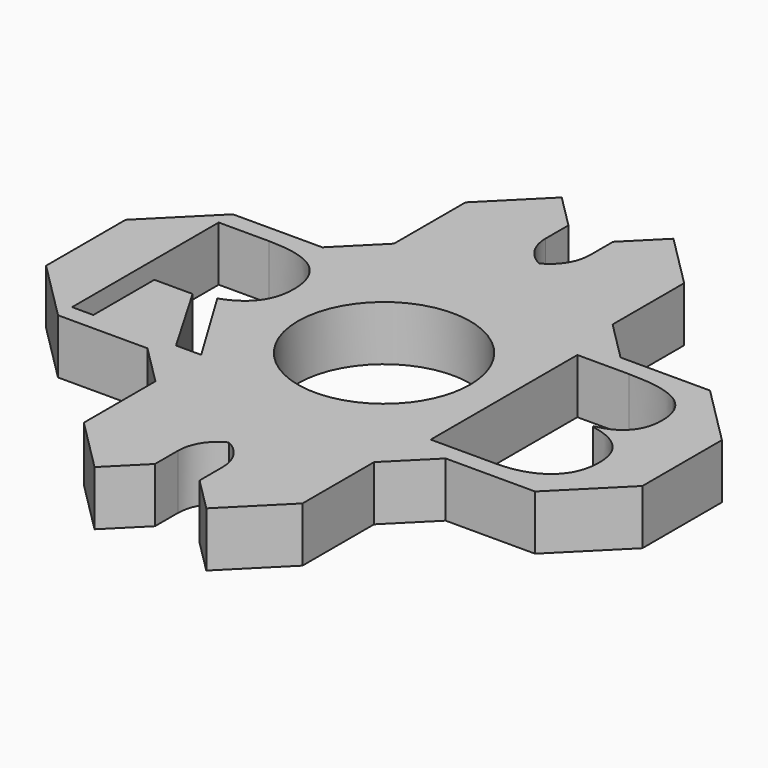
from build123d import *

# Parameters (mm, degrees)
F0_W        = 24.13
F0_H        = 27.94
F0_W_2      = 27.94
F1_DEPTH    = 7
F0_H_2      = 24.13
F2_DEPTH    = 7
F3_SIZE     = 7.62
F4_SIZE     = 5.08
F5_W        = 5.6953141466
F5_H        = 27.5579802692
F5_H_2      = 20.2091857791
F6_DEPTH    = 46.736
F7_T1_DEPTH = 33.1282991577
F8_T1_DEPTH = 7


# Not quite as in the source:
# - a fillet or chamfer that OpenCascade refuses, or shapes differently, is made with other operations: its cross-section is extruded or revolved along the edge and cut away or added


with BuildPart() as f1:
    # F0 (on Top) → F1 (new body)
    with BuildSketch(Plane.XY):
        with Locations((-26.035, 0)):
            Rectangle(F0_W, F0_H)
        with BuildLine():
            Line((-22.8701785602, -1.9821503455), (-27.7604957957, -1.9821503455))
            Line((-27.7604957957, -1.9821503455), (-27.7604957957, -11.721775867))
            Line((-27.7604957957, -11.721775867), (-30.4824648231, -11.721775867))
            Line((-30.4824648231, -11.721775867), (-30.4824648231, 11.6994604529))
            Line((-30.4824648231, 11.6994604529), (-24.0594380975, 11.6994604529))
            add(Edge.make_bspline(
                [(-24.0594380975, 11.6994604529), (-19.7483722746, 11.6994604529), (-17.6902356183, 10.0488502329)],
                knots=[0, 0, 0, 1, 1, 1], degree=2))
            add(Edge.make_bspline(
                [(-17.6902356183, 10.0488502329), (-15.6320989621, 8.398240013), (-15.6320989621, 5.0816412169)],
                knots=[0, 0, 0, 1, 1, 1], degree=2))
            add(Edge.make_bspline(
                [(-15.6320989621, 5.0816412169), (-15.6320989621, 0.4373776788), (-20.3430020433, -1.1978541851)],
                knots=[0, 0, 0, 1, 1, 1], degree=2))
            Line((-20.3430020433, -1.1978541851), (-13.9814887421, -11.721775867))
            Line((-13.9814887421, -11.721775867), (-17.2006912829, -11.721775867))
            Line((-17.2006912829, -11.721775867), (-22.8701785602, -1.9821503455))
        make_face(mode=Mode.SUBTRACT)
        Rectangle(F0_W_2, F0_H)
        with BuildLine():
            ThreePointArc((8.7965986845, 6.6045326545), (10.4346199147, 3.4811933637), (11, 0))
            ThreePointArc((11, 0), (10.4117353498, -3.5490515643), (8.7098605443, -6.7185064783))
            add(Edge.make_bspline(
                [(8.7098605443, -6.7185064783), (8.1189739543, -7.8747447622), (7.281651607, -8.8229557447)],
                knots=[0.7056859188, 0.7056859188, 0.7056859188, 1, 1, 1], degree=2))
            add(Edge.make_bspline(
                [(7.281651607, -8.8229557447), (4.436655731, -12.0447213449), (-0.6228234215, -12.0447213449)],
                knots=[0, 0, 0, 1, 1, 1], degree=2))
            add(Edge.make_bspline(
                [(-0.6228234215, -12.0447213449), (-5.7950771853, -12.0447213449), (-8.6067532898, -8.8793430504)],
                knots=[0, 0, 0, 1, 1, 1], degree=2))
            add(Edge.make_bspline(
                [(-8.6067532898, -8.8793430504), (-11.4184293943, -5.7139647559), (-11.4184293943, 0.0529187766)],
                knots=[0, 0, 0, 1, 1, 1], degree=2))
            add(Edge.make_bspline(
                [(-11.4184293943, 0.0529187766), (-11.4184293943, 5.7736672408), (-8.5990641118, 8.9211041199)],
                knots=[0, 0, 0, 1, 1, 1], degree=2))
            add(Edge.make_bspline(
                [(-8.5990641118, 8.9211041199), (-5.7796988292, 12.068540999), (-0.5920667093, 12.068540999)],
                knots=[0, 0, 0, 1, 1, 1], degree=2))
            add(Edge.make_bspline(
                [(-0.5920667093, 12.068540999), (4.4571602058, 12.068540999), (7.2919038444, 8.8647168143)],
                knots=[0, 0, 0, 1, 1, 1], degree=2))
            add(Edge.make_bspline(
                [(7.2919038444, 8.8647168143), (8.1849092487, 7.8554430753), (8.7965986845, 6.6045326545)],
                knots=[0, 0, 0, 0.3150215745, 0.3150215745, 0.3150215745], degree=2))
        make_face(mode=Mode.SUBTRACT)
        with Locations((26.035, 0)):
            Rectangle(F0_W, F0_H)
        with BuildLine():
            Line((15.3450363151, -11.721775867), (15.3450363151, 11.6994604529))
            Line((15.3450363151, 11.6994604529), (21.9628555511, 11.6994604529))
            add(Edge.make_bspline(
                [(21.9628555511, 11.6994604529), (26.6224974453, 11.6994604529), (28.706264695, 10.3051561677)],
                knots=[0, 0, 0, 1, 1, 1], degree=2))
            add(Edge.make_bspline(
                [(28.706264695, 10.3051561677), (30.7900319448, 8.9108518825), (30.7900319448, 5.9018202082)],
                knots=[0, 0, 0, 1, 1, 1], degree=2))
            add(Edge.make_bspline(
                [(30.7900319448, 5.9018202082), (30.7900319448, 3.8154898992), (29.6289660602, 2.4621945635)],
                knots=[0, 0, 0, 1, 1, 1], degree=2))
            add(Edge.make_bspline(
                [(29.6289660602, 2.4621945635), (28.4679001757, 1.1088992279), (26.2380385431, 0.7090619697)],
                knots=[0, 0, 0, 1, 1, 1], degree=2))
            Line((26.2380385431, 0.7090619697), (26.2380385431, 0.5501522901))
            add(Edge.make_bspline(
                [(26.2380385431, 0.5501522901), (31.5743281052, -0.3622968377), (31.5743281052, -5.0578215628)],
                knots=[0, 0, 0, 1, 1, 1], degree=2))
            add(Edge.make_bspline(
                [(31.5743281052, -5.0578215628), (31.5743281052, -8.1950062045), (29.4521149653, -9.9583910358)],
                knots=[0, 0, 0, 1, 1, 1], degree=2))
            add(Edge.make_bspline(
                [(29.4521149653, -9.9583910358), (27.3299018253, -11.721775867), (23.5160695158, -11.721775867)],
                knots=[0, 0, 0, 1, 1, 1], degree=2))
            Line((23.5160695158, -11.721775867), (15.3450363151, -11.721775867))
        make_face(mode=Mode.SUBTRACT)
        with BuildLine():
            ThreePointArc((8.7098605443, -6.7185064783), (-10.9997668891, 0.0716127389), (8.7965986845, 6.6045326545))
            add(Edge.make_bspline(
                [(7.2919038444, 8.8647168143), (8.1849092487, 7.8554430753), (8.7965986845, 6.6045326545)],
                knots=[0, 0, 0, 0.3150215745, 0.3150215745, 0.3150215745], degree=2))
            add(Edge.make_bspline(
                [(-0.5920667093, 12.068540999), (4.4571602058, 12.068540999), (7.2919038444, 8.8647168143)],
                knots=[0, 0, 0, 1, 1, 1], degree=2))
            add(Edge.make_bspline(
                [(-8.5990641118, 8.9211041199), (-5.7796988292, 12.068540999), (-0.5920667093, 12.068540999)],
                knots=[0, 0, 0, 1, 1, 1], degree=2))
            add(Edge.make_bspline(
                [(-11.4184293943, 0.0529187766), (-11.4184293943, 5.7736672408), (-8.5990641118, 8.9211041199)],
                knots=[0, 0, 0, 1, 1, 1], degree=2))
            add(Edge.make_bspline(
                [(-8.6067532898, -8.8793430504), (-11.4184293943, -5.7139647559), (-11.4184293943, 0.0529187766)],
                knots=[0, 0, 0, 1, 1, 1], degree=2))
            add(Edge.make_bspline(
                [(-0.6228234215, -12.0447213449), (-5.7950771853, -12.0447213449), (-8.6067532898, -8.8793430504)],
                knots=[0, 0, 0, 1, 1, 1], degree=2))
            add(Edge.make_bspline(
                [(7.281651607, -8.8229557447), (4.436655731, -12.0447213449), (-0.6228234215, -12.0447213449)],
                knots=[0, 0, 0, 1, 1, 1], degree=2))
            add(Edge.make_bspline(
                [(8.7098605443, -6.7185064783), (8.1189739543, -7.8747447622), (7.281651607, -8.8229557447)],
                knots=[0.7056859188, 0.7056859188, 0.7056859188, 1, 1, 1], degree=2))
        make_face()
    extrude(amount=F1_DEPTH)

    # F0 (on Top) → F2 (join)
    with BuildSketch(Plane.XY):
        with Locations((-26.035, 0)):
            Rectangle(F0_W, F0_H)
        with BuildLine():
            Line((-22.8701785602, -1.9821503455), (-27.7604957957, -1.9821503455))
            Line((-27.7604957957, -1.9821503455), (-27.7604957957, -11.721775867))
            Line((-27.7604957957, -11.721775867), (-30.4824648231, -11.721775867))
            Line((-30.4824648231, -11.721775867), (-30.4824648231, 11.6994604529))
            Line((-30.4824648231, 11.6994604529), (-24.0594380975, 11.6994604529))
            add(Edge.make_bspline(
                [(-24.0594380975, 11.6994604529), (-19.7483722746, 11.6994604529), (-17.6902356183, 10.0488502329)],
                knots=[0, 0, 0, 1, 1, 1], degree=2))
            add(Edge.make_bspline(
                [(-17.6902356183, 10.0488502329), (-15.6320989621, 8.398240013), (-15.6320989621, 5.0816412169)],
                knots=[0, 0, 0, 1, 1, 1], degree=2))
            add(Edge.make_bspline(
                [(-15.6320989621, 5.0816412169), (-15.6320989621, 0.4373776788), (-20.3430020433, -1.1978541851)],
                knots=[0, 0, 0, 1, 1, 1], degree=2))
            Line((-20.3430020433, -1.1978541851), (-13.9814887421, -11.721775867))
            Line((-13.9814887421, -11.721775867), (-17.2006912829, -11.721775867))
            Line((-17.2006912829, -11.721775867), (-22.8701785602, -1.9821503455))
        make_face(mode=Mode.SUBTRACT)
        Rectangle(F0_W_2, F0_H)
        with BuildLine():
            ThreePointArc((8.7965986845, 6.6045326545), (10.4346199147, 3.4811933637), (11, 0))
            ThreePointArc((11, 0), (10.4117353498, -3.5490515643), (8.7098605443, -6.7185064783))
            add(Edge.make_bspline(
                [(8.7098605443, -6.7185064783), (8.1189739543, -7.8747447622), (7.281651607, -8.8229557447)],
                knots=[0.7056859188, 0.7056859188, 0.7056859188, 1, 1, 1], degree=2))
            add(Edge.make_bspline(
                [(7.281651607, -8.8229557447), (4.436655731, -12.0447213449), (-0.6228234215, -12.0447213449)],
                knots=[0, 0, 0, 1, 1, 1], degree=2))
            add(Edge.make_bspline(
                [(-0.6228234215, -12.0447213449), (-5.7950771853, -12.0447213449), (-8.6067532898, -8.8793430504)],
                knots=[0, 0, 0, 1, 1, 1], degree=2))
            add(Edge.make_bspline(
                [(-8.6067532898, -8.8793430504), (-11.4184293943, -5.7139647559), (-11.4184293943, 0.0529187766)],
                knots=[0, 0, 0, 1, 1, 1], degree=2))
            add(Edge.make_bspline(
                [(-11.4184293943, 0.0529187766), (-11.4184293943, 5.7736672408), (-8.5990641118, 8.9211041199)],
                knots=[0, 0, 0, 1, 1, 1], degree=2))
            add(Edge.make_bspline(
                [(-8.5990641118, 8.9211041199), (-5.7796988292, 12.068540999), (-0.5920667093, 12.068540999)],
                knots=[0, 0, 0, 1, 1, 1], degree=2))
            add(Edge.make_bspline(
                [(-0.5920667093, 12.068540999), (4.4571602058, 12.068540999), (7.2919038444, 8.8647168143)],
                knots=[0, 0, 0, 1, 1, 1], degree=2))
            add(Edge.make_bspline(
                [(7.2919038444, 8.8647168143), (8.1849092487, 7.8554430753), (8.7965986845, 6.6045326545)],
                knots=[0, 0, 0, 0.3150215745, 0.3150215745, 0.3150215745], degree=2))
        make_face(mode=Mode.SUBTRACT)
        with BuildLine():
            ThreePointArc((8.7098605443, -6.7185064783), (-10.9997668891, 0.0716127389), (8.7965986845, 6.6045326545))
            add(Edge.make_bspline(
                [(7.2919038444, 8.8647168143), (8.1849092487, 7.8554430753), (8.7965986845, 6.6045326545)],
                knots=[0, 0, 0, 0.3150215745, 0.3150215745, 0.3150215745], degree=2))
            add(Edge.make_bspline(
                [(-0.5920667093, 12.068540999), (4.4571602058, 12.068540999), (7.2919038444, 8.8647168143)],
                knots=[0, 0, 0, 1, 1, 1], degree=2))
            add(Edge.make_bspline(
                [(-8.5990641118, 8.9211041199), (-5.7796988292, 12.068540999), (-0.5920667093, 12.068540999)],
                knots=[0, 0, 0, 1, 1, 1], degree=2))
            add(Edge.make_bspline(
                [(-11.4184293943, 0.0529187766), (-11.4184293943, 5.7736672408), (-8.5990641118, 8.9211041199)],
                knots=[0, 0, 0, 1, 1, 1], degree=2))
            add(Edge.make_bspline(
                [(-8.6067532898, -8.8793430504), (-11.4184293943, -5.7139647559), (-11.4184293943, 0.0529187766)],
                knots=[0, 0, 0, 1, 1, 1], degree=2))
            add(Edge.make_bspline(
                [(-0.6228234215, -12.0447213449), (-5.7950771853, -12.0447213449), (-8.6067532898, -8.8793430504)],
                knots=[0, 0, 0, 1, 1, 1], degree=2))
            add(Edge.make_bspline(
                [(7.281651607, -8.8229557447), (4.436655731, -12.0447213449), (-0.6228234215, -12.0447213449)],
                knots=[0, 0, 0, 1, 1, 1], degree=2))
            add(Edge.make_bspline(
                [(8.7098605443, -6.7185064783), (8.1189739543, -7.8747447622), (7.281651607, -8.8229557447)],
                knots=[0.7056859188, 0.7056859188, 0.7056859188, 1, 1, 1], degree=2))
        make_face()
        with Locations((26.035, 0)):
            Rectangle(F0_W, F0_H)
        with BuildLine():
            Line((15.3450363151, -11.721775867), (15.3450363151, 11.6994604529))
            Line((15.3450363151, 11.6994604529), (21.9628555511, 11.6994604529))
            add(Edge.make_bspline(
                [(21.9628555511, 11.6994604529), (26.6224974453, 11.6994604529), (28.706264695, 10.3051561677)],
                knots=[0, 0, 0, 1, 1, 1], degree=2))
            add(Edge.make_bspline(
                [(28.706264695, 10.3051561677), (30.7900319448, 8.9108518825), (30.7900319448, 5.9018202082)],
                knots=[0, 0, 0, 1, 1, 1], degree=2))
            add(Edge.make_bspline(
                [(30.7900319448, 5.9018202082), (30.7900319448, 3.8154898992), (29.6289660602, 2.4621945635)],
                knots=[0, 0, 0, 1, 1, 1], degree=2))
            add(Edge.make_bspline(
                [(29.6289660602, 2.4621945635), (28.4679001757, 1.1088992279), (26.2380385431, 0.7090619697)],
                knots=[0, 0, 0, 1, 1, 1], degree=2))
            Line((26.2380385431, 0.7090619697), (26.2380385431, 0.5501522901))
            add(Edge.make_bspline(
                [(26.2380385431, 0.5501522901), (31.5743281052, -0.3622968377), (31.5743281052, -5.0578215628)],
                knots=[0, 0, 0, 1, 1, 1], degree=2))
            add(Edge.make_bspline(
                [(31.5743281052, -5.0578215628), (31.5743281052, -8.1950062045), (29.4521149653, -9.9583910358)],
                knots=[0, 0, 0, 1, 1, 1], degree=2))
            add(Edge.make_bspline(
                [(29.4521149653, -9.9583910358), (27.3299018253, -11.721775867), (23.5160695158, -11.721775867)],
                knots=[0, 0, 0, 1, 1, 1], degree=2))
            Line((23.5160695158, -11.721775867), (15.3450363151, -11.721775867))
        make_face(mode=Mode.SUBTRACT)
        with Locations((0, 26.035)):
            Rectangle(F0_W_2, F0_H_2)
        with Locations((0, -26.035)):
            Rectangle(F0_W_2, F0_H_2)
    extrude(amount=F2_DEPTH)

    # F3
    f3_edges = [f1.edges().sort_by_distance(p)[0] for p in [
        (13.97, 38.1, 3.5),
        (-13.97, 38.1, 3.5),
        (13.97, -38.1, 3.5),
        (-13.97, -38.1, 3.5),
        (38.1, -13.97, 3.5),
        (38.1, 13.97, 3.5),
        (-38.1, -13.97, 3.5),
        (-38.1, 13.97, 3.5),
    ]]
    chamfer(f3_edges, length=F3_SIZE)

    # F4
    f4_edges = [f1.edges().sort_by_distance(p)[0] for p in [
        (-13.97, -13.97, 3.5),
        (13.97, -13.97, 3.5),
        (-13.97, 13.97, 3.5),
        (13.97, 13.97, 3.5),
    ]]
    chamfer(f4_edges, length=F4_SIZE)

    # F5 (on Top) → F6 (cut)
    with BuildSketch(Plane.XY):
        with Locations((0, 38.0300115794)):
            Rectangle(F5_W, F5_H)
        with Locations((0, -34.3556143343)):
            Rectangle(F5_W, F5_H_2)
    extrude(amount=F6_DEPTH, mode=Mode.SUBTRACT)

    # F7: chamfer of 5.08 on 4 edges, made by hand

    # F7_s2 → F7_t1 (cut)
    with BuildSketch(Plane.XY.offset(-13.0641495789)):
        Polygon((2.8476570733, 33.02), (7.9276570733, 38.1), (2.8476570733, 38.1), align=None)
        Polygon((-7.9276570733, 38.1), (-2.8476570733, 33.02), (-2.8476570733, 38.1), align=None)
        Polygon((-2.8476570733, -33.02), (-7.9276570733, -38.1), (-2.8476570733, -38.1), align=None)
        Polygon((7.9276570733, -38.1), (2.8476570733, -33.02), (2.8476570733, -38.1), align=None)
    extrude(amount=F7_T1_DEPTH, mode=Mode.SUBTRACT)

    # F8: fillet of radius 5.08 on 4 edges, made by hand

    # F8_s2 → F8_t1 (join)
    with BuildSketch(Plane.XY):
        with BuildLine():
            ThreePointArc((-2.2323429267, 24.2510214448), (1.3597595217, 25.7389189964), (2.8476570733, 29.3310214448))
            Line((2.8476570733, 29.3310214448), (2.8476570733, 24.2510214448))
            Line((2.8476570733, 24.2510214448), (-2.2323429267, 24.2510214448))
        make_face()
        with BuildLine():
            ThreePointArc((-2.8476570733, 29.3310214448), (-1.3597595217, 25.7389189964), (2.2323429267, 24.2510214448))
            Line((2.2323429267, 24.2510214448), (-2.8476570733, 24.2510214448))
            Line((-2.8476570733, 24.2510214448), (-2.8476570733, 29.3310214448))
        make_face()
        with BuildLine():
            ThreePointArc((2.8476570733, -29.3310214448), (1.3597595217, -25.7389189964), (-2.2323429267, -24.2510214448))
            Line((-2.2323429267, -24.2510214448), (2.8476570733, -24.2510214448))
            Line((2.8476570733, -24.2510214448), (2.8476570733, -29.3310214448))
        make_face()
        with BuildLine():
            ThreePointArc((2.2323429267, -24.2510214448), (-1.3597595217, -25.7389189964), (-2.8476570733, -29.3310214448))
            Line((-2.8476570733, -29.3310214448), (-2.8476570733, -24.2510214448))
            Line((-2.8476570733, -24.2510214448), (2.2323429267, -24.2510214448))
        make_face()
    extrude(amount=F8_T1_DEPTH)


solid = f1.part
